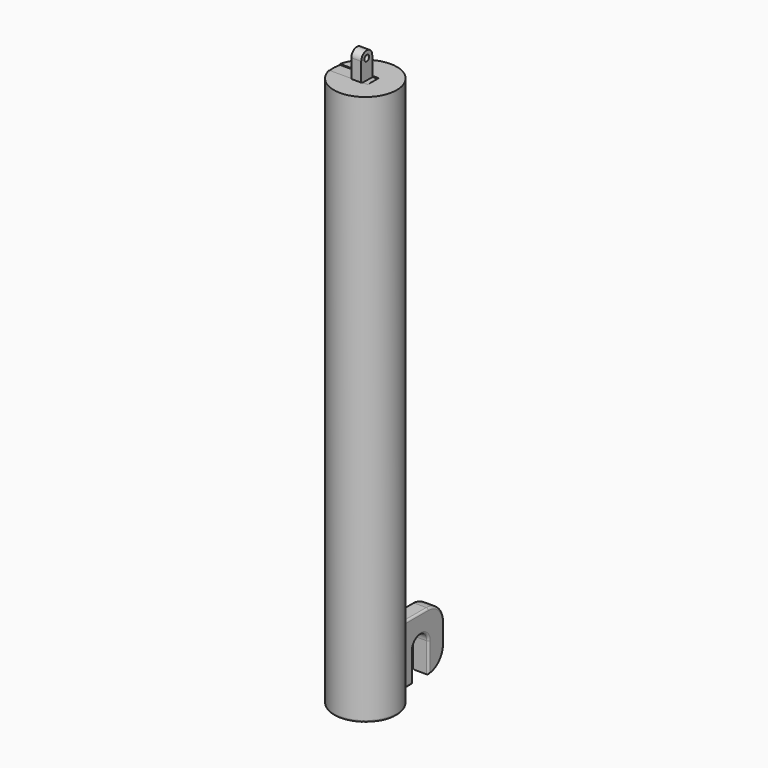
from build123d import *

# Parameters (mm, degrees)
F0_R        = 16
F1_DEPTH    = 280
F2_W        = 45
F2_H        = 30
F3_DEPTH    = 4
F4_R        = 1.5
F5_DEPTH    = 25
F6_T1_DEPTH = 58
F6_T3_DEPTH = 57.9848728082
F7_R        = 1
F9_DEPTH    = 5


# Not quite as in the source:
# - a fillet or chamfer that OpenCascade refuses, or shapes differently, is made with other operations: its cross-section is extruded or revolved along the edge and cut away or added


with BuildPart() as f1:
    # F0 (on Top) → F1 (new body)
    with BuildSketch(Plane.XY):
        Circle(F0_R)
    extrude(amount=F1_DEPTH)

    # F2 (on Right) → F3 (join, symmetric)
    with BuildSketch(Plane.YZ):
        with Locations((22.5, 15)):
            Rectangle(F2_W, F2_H)
    extrude(amount=F3_DEPTH, both=True)

    # F4 (on face) → F5 (cut)
    with BuildSketch(Plane.YZ.offset(4)):
        with BuildLine():
            ThreePointArc((25.2459666924, 15), (30.2459666924, 10), (35.2459666924, 15))
            ThreePointArc((35.2459666924, 15), (30.2459666924, 20), (25.2459666924, 15))
        make_face()
        with BuildLine():
            ThreePointArc((-3.5, 286.5642011166), (0, 283.0642011166), (3.5, 286.5642011166))
            ThreePointArc((3.5, 286.5642011166), (0, 290.0642011166), (-3.5, 286.5642011166))
        make_face()
        with Locations((0, 286.5642011166)):
            Circle(F4_R, mode=Mode.SUBTRACT)
        with BuildLine():
            Line((3.5, 279.5200645924), (3.5, 286.5642011166))
            ThreePointArc((3.5, 286.5642011166), (0, 283.0642011166), (-3.5, 286.5642011166))
            Line((-3.5, 286.5642011166), (-3.5, 279.665210771))
            Line((-3.5, 279.665210771), (3.5, 279.5200645924))
        make_face()
        with BuildLine():
            Line((35.2459666924, 0), (35.2459666924, 15))
            ThreePointArc((35.2459666924, 15), (30.2459666924, 10), (25.2459666924, 15))
            Line((25.2459666924, 15), (25.2459666924, 0))
            Line((25.2459666924, 0), (35.2459666924, 0))
        make_face()
    extrude(amount=-F5_DEPTH, mode=Mode.SUBTRACT)

    # F6: fillet of radius 10 on 2 edges, made by hand

    # F6_s2 → F6_t1 (cut)
    with BuildSketch(Plane.YZ.offset(-29)):
        with BuildLine():
            ThreePointArc((35, 30), (42.0710678119, 27.0710678119), (45, 20))
            Line((45, 20), (45, 30))
            Line((45, 30), (35, 30))
        make_face()
    extrude(amount=F6_T1_DEPTH, mode=Mode.SUBTRACT)

    # F6_s4 → F6_t3 (cut)
    with BuildSketch(Plane.YZ.offset(-28.9924364041)):
        with BuildLine():
            ThreePointArc((35.2459666924, 0), (42.1575019009, 3.0134105333), (45, 9.9969745616))
            Line((45, 9.9969745616), (45, 0))
            Line((45, 0), (35.2459666924, 0))
        make_face()
    extrude(amount=F6_T3_DEPTH, mode=Mode.SUBTRACT)

    # F7
    f7_edges = [f1.edges().sort_by_distance(p)[0] for p in [
        (4, 42.071068, 27.071068),
        (-4, 45, 14.998487),
        (4, 35.245967, 7.5),
        (4, 30.245967, 20),
        (4, 25.245967, 7.5),
        (4, 20.36895, 0),
        (4, 15.491933, 15),
        (4, 25.245967, 30),
        (4, 45, 14.998487),
        (4, 42.157502, 3.013411),
        (12.649111, 9.797959, 0),
        (0, 16, 30),
        (-4, 15.491933, 15),
        (-9.797959, -12.649111, 0),
        (-4, 20.36895, 0),
        (-4, 25.245967, 30),
        (-4, 42.071068, 27.071068),
        (-4, 42.157502, 3.013411),
    ]]
    fillet(f7_edges, radius=F7_R)

    # F8 (on face) → F9 (join)
    with BuildSketch(Plane(origin=(-4, 0, 0), x_dir=(0, -1, 0), z_dir=(-1, 0, 0))):
        with BuildLine():
            Line((-3.1555609312, 289.529184103), (-3.1555609312, 279.529184103))
            Line((-3.1555609312, 279.529184103), (3.8444390688, 279.529184103))
            Line((3.8444390688, 279.529184103), (3.8444390688, 289.529184103))
            ThreePointArc((3.8444390688, 289.529184103), (0.3444390688, 286.029184103), (-3.1555609312, 289.529184103))
        make_face()
        with BuildLine():
            ThreePointArc((3.8444390688, 289.529184103), (0.3444390688, 293.029184103), (-3.1555609312, 289.529184103))
            Line((-3.1555609312, 289.529184103), (-1.1555609312, 289.529184103))
            ThreePointArc((-1.1555609312, 289.529184103), (0.3444390688, 291.029184103), (1.8444390688, 289.529184103))
            Line((1.8444390688, 289.529184103), (3.8444390688, 289.529184103))
        make_face()
        with BuildLine():
            Line((-1.1555609312, 289.529184103), (-3.1555609312, 289.529184103))
            ThreePointArc((-3.1555609312, 289.529184103), (0.3444390688, 286.029184103), (3.8444390688, 289.529184103))
            Line((3.8444390688, 289.529184103), (1.8444390688, 289.529184103))
            ThreePointArc((1.8444390688, 289.529184103), (0.3444390688, 288.029184103), (-1.1555609312, 289.529184103))
        make_face()
    extrude(amount=-F9_DEPTH)


solid = f1.part
